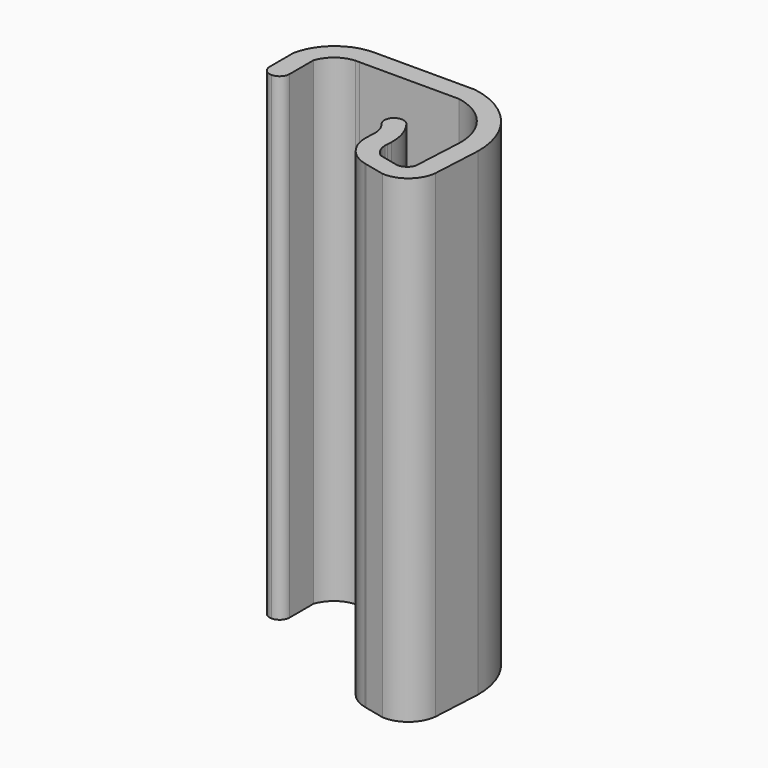
from build123d import *

# Parameters (mm, degrees)
F1_DEPTH    = 48
F2_SIZE     = 6
F3_T1_DEPTH = 53
F3_T3_DEPTH = 54.5281651471
F3_T5_DEPTH = 52.4600037496


# Not quite as in the source:
# - a fillet or chamfer that OpenCascade refuses, or shapes differently, is made with other operations: its cross-section is extruded or revolved along the edge and cut away or added
# - a feature names something its author has since deleted; it is built from what else it names


with BuildPart() as f1:
    # F0 (on Top) → F1 (new body)
    with BuildSketch(Plane.XY):
        with BuildLine():
            Line((0, 4), (0, 0))
            Line((0, 0), (2, 0))
            Line((2, 0), (2, 4))
            ThreePointArc((2, 4), (3.0020118724, 5.3950578705), (4.6095750202, 6))
            ThreePointArc((4.6095750202, 6), (4.8047875101, 6.0064362795), (5, 6))
            Line((5, 6), (15, 6))
            ThreePointArc((15, 6), (18.4461762663, 3.9255722455), (19.6880345723, 0.0997168751))
            ThreePointArc((19.6880345723, 0.0997168751), (19.6856381883, 0.0498470868), (19.6828086323, 0))
            Line((19.6828086323, 0), (19.4207697359, -5))
            ThreePointArc((19.4207697359, -5), (18.9661763427, -5.5793756098), (18.26629109, -5.8084866821))
            Line((18.26629109, -5.8084866821), (16.1894012844, -5.3289988895))
            ThreePointArc((16.1894012844, -5.3289988895), (15.6261580996, -4.6575642289), (15.4106099526, -3.8080900476))
            ThreePointArc((15.4106099526, -3.8080900476), (15.4127500759, -3.6584901874), (15.4262591199, -3.5094861471))
            Line((15.4262591199, -3.5094861471), (15.4524630095, -3.0094861471))
            ThreePointArc((15.4524630095, -3.0094861471), (14.9662231771, -0.7637354985), (13.5283299865, 1.0285502831))
            Line((13.5283299865, 1.0285502831), (12.346313856, -0.5859939341))
            ThreePointArc((12.346313856, -0.5859939341), (12.5114130289, -0.7045010308), (12.6663410631, -0.8360265911))
            ThreePointArc((12.6663410631, -0.8360265911), (13.2467923067, -1.6369828382), (13.4711592073, -2.6003695984))
            ThreePointArc((13.4711592073, -2.6003695984), (13.4688331774, -2.8053678054), (13.4497183175, -3.0094861471))
            Line((13.4497183175, -3.0094861471), (13.4235144279, -3.5094861471))
            Line((13.4235144279, -3.5094861471), (13.4164237789, -3.6447837895))
            ThreePointArc((13.4164237789, -3.6447837895), (14.1205058655, -5.8682370303), (16.0652377732, -7.1556739049))
            Line((16.0652377732, -7.1556739049), (16.1894012844, -7.1843393101))
            Line((16.1894012844, -7.1843393101), (18.26629109, -7.6638271027))
            ThreePointArc((18.26629109, -7.6638271027), (20.3764129686, -6.9618705168), (21.4235144279, -5))
            Line((21.4235144279, -5), (21.6855533243, 0))
            ThreePointArc((21.6855533243, 0), (19.8249274325, 5.2386247512), (15, 8))
            Line((15, 8), (7, 8))
            Line((7, 8), (7, 14))
            Line((7, 14), (5, 14))
            Line((5, 14), (5, 8))
            Line((5, 8), (4.7983737082, 8))
            ThreePointArc((4.7983737082, 8), (1.6976247354, 6.8415893063), (0, 4))
        make_face()
    extrude(amount=F1_DEPTH)

    # F2
    f2_edges = [f1.edges().sort_by_distance(p)[0] for p in [
        (6, 14, 48),
        (6, 14, 0),
    ]]
    chamfer(f2_edges, length=F2_SIZE)

    # F3: fillet of radius 1 on 4 edges, made by hand

    # F3_s2 → F3_t1 (cut)
    with BuildSketch(Plane.XY.offset(-2.5)):
        with BuildLine():
            ThreePointArc((0, 1), (0.2928932188, 0.2928932188), (1, 0))
            Line((1, 0), (0, 0))
            Line((0, 0), (0, 1))
        make_face()
        with BuildLine():
            ThreePointArc((1, 0), (1.7071067812, 0.2928932188), (2, 1))
            Line((2, 1), (2, 0))
            Line((2, 0), (1, 0))
        make_face()
    extrude(amount=F3_T1_DEPTH, mode=Mode.SUBTRACT)

    # F3_s4 → F3_t3 (cut)
    with BuildSketch(Plane.XY.offset(-3.2640825735)):
        with BuildLine():
            ThreePointArc((12.8383454605, 0.0860838499), (13.6381253577, 0.495339622), (14.4436338584, 0.0974775525))
            ThreePointArc((14.4436338584, 0.0974775525), (14.0164512092, 0.5929671699), (13.5283299865, 1.0285502831))
            Line((13.5283299865, 1.0285502831), (12.8383454605, 0.0860838499))
        make_face()
    extrude(amount=F3_T3_DEPTH, mode=Mode.SUBTRACT)

    # F3_s6 → F3_t5 (cut)
    with BuildSketch(Plane.XY.offset(-2.2300018748)):
        with BuildLine():
            ThreePointArc((12.9064405307, -1.0905635453), (12.6804805888, -0.4840892178), (12.8732356835, 0.1337412433))
            Line((12.8732356835, 0.1337412433), (12.346313856, -0.5859939341))
            ThreePointArc((12.346313856, -0.5859939341), (12.6455057343, -0.8170439967), (12.9064405307, -1.0905635453))
        make_face()
    extrude(amount=F3_T5_DEPTH, mode=Mode.SUBTRACT)


solid = f1.part
